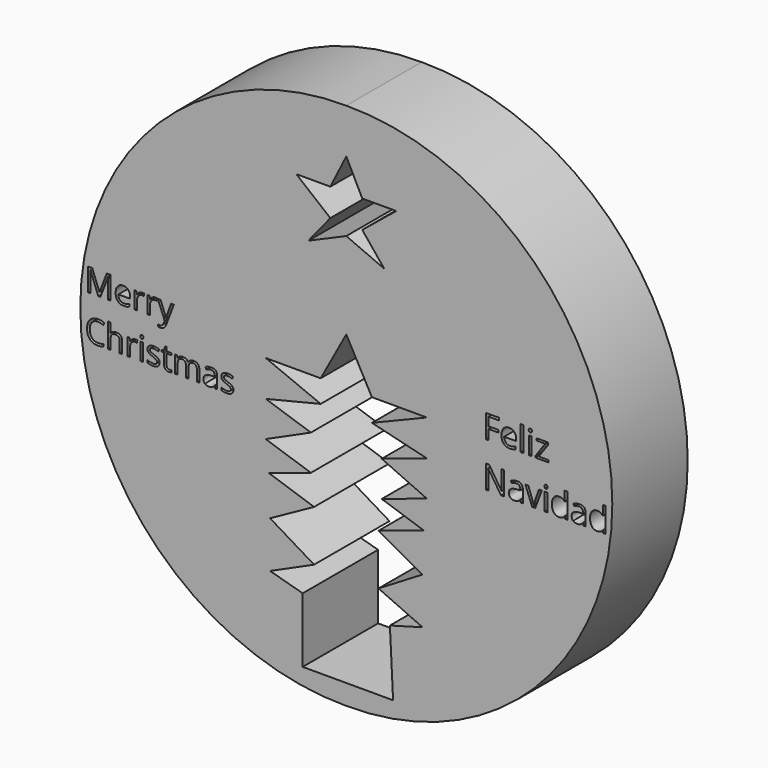
from build123d import *

# Parameters (mm, degrees)
F0_W     = 0.6967988684
F0_H     = 4.5983354994
F0_W_2   = 0.7130679342
F0_H_2   = 4.7056987948
F0_H_3   = 6.6814053253
F1_DEPTH = 25.4


with BuildPart() as f1:
    # F0 (on Front) → F1 (new body)
    with BuildSketch(Plane.XZ):
        with BuildLine():
            ThreePointArc((0, -75.4838734865), (71.6859873909, -4.2729414999), (0, 66.9379904866))
            ThreePointArc((0, 66.9379904866), (-71.6859873909, -4.2729414999), (0, -75.4838734865))
        make_face()
        with BuildLine():
            add(Edge.make_bspline(
                [(-65.5339630569, -6.4282716412), (-66.2307619253, -6.1020247722), (-66.9275607937, -6.1020247722)],
                knots=[0, 0, 0, 1, 1, 1], degree=2))
            add(Edge.make_bspline(
                [(-66.9275607937, -6.1020247722), (-67.9385233137, -6.1020247722), (-68.5238880663, -6.7753284957)],
                knots=[0, 0, 0, 1, 1, 1], degree=2))
            add(Edge.make_bspline(
                [(-68.5238880663, -6.7753284957), (-69.1092528189, -7.4486322192), (-69.1092528189, -8.6193617244)],
                knots=[0, 0, 0, 1, 1, 1], degree=2))
            add(Edge.make_bspline(
                [(-69.1092528189, -8.6193617244), (-69.1092528189, -9.8223131426), (-68.5446980518, -10.4795059096)],
                knots=[0, 0, 0, 1, 1, 1], degree=2))
            add(Edge.make_bspline(
                [(-68.5446980518, -10.4795059096), (-67.9801432846, -11.1366986766), (-66.9356162719, -11.1366986766)],
                knots=[0, 0, 0, 1, 1, 1], degree=2))
            add(Edge.make_bspline(
                [(-66.9356162719, -11.1366986766), (-66.2938631716, -11.1366986766), (-65.4708618106, -10.9057749669)],
                knots=[0, 0, 0, 1, 1, 1], degree=2))
            Line((-65.4708618106, -10.9057749669), (-65.4708618106, -11.530074531))
            add(Edge.make_bspline(
                [(-65.4708618106, -11.530074531), (-66.1085871719, -11.7703962987), (-67.0443652283, -11.7703962987)],
                knots=[0, 0, 0, 1, 1, 1], degree=2))
            add(Edge.make_bspline(
                [(-67.0443652283, -11.7703962987), (-68.3990281535, -11.7703962987), (-69.1354331232, -10.9473949378)],
                knots=[0, 0, 0, 1, 1, 1], degree=2))
            add(Edge.make_bspline(
                [(-69.1354331232, -10.9473949378), (-69.871838093, -10.1243935769), (-69.871838093, -8.6099636665)],
                knots=[0, 0, 0, 1, 1, 1], degree=2))
            add(Edge.make_bspline(
                [(-69.871838093, -8.6099636665), (-69.871838093, -7.6621023927), (-69.5173970501, -6.9491925678)],
                knots=[0, 0, 0, 1, 1, 1], degree=2))
            add(Edge.make_bspline(
                [(-69.5173970501, -6.9491925678), (-69.1629560072, -6.236282743), (-68.4936800229, -5.850291077)],
                knots=[0, 0, 0, 1, 1, 1], degree=2))
            add(Edge.make_bspline(
                [(-68.4936800229, -5.850291077), (-67.8244040385, -5.464299411), (-66.9181627357, -5.464299411)],
                knots=[0, 0, 0, 1, 1, 1], degree=2))
            add(Edge.make_bspline(
                [(-66.9181627357, -5.464299411), (-65.9541905055, -5.464299411), (-65.2318826227, -5.8160552944)],
                knots=[0, 0, 0, 1, 1, 1], degree=2))
            Line((-65.2318826227, -5.8160552944), (-65.5339630569, -6.4282716412))
        make_face(mode=Mode.SUBTRACT)
        with BuildLine():
            add(Edge.make_bspline(
                [(-57.6583904907, -7.2465739731), (-57.2972365492, -7.0028957562), (-56.8649258833, -7.0028957562)],
                knots=[0, 0, 0, 1, 1, 1], degree=2))
            add(Edge.make_bspline(
                [(-56.8649258833, -7.0028957562), (-56.5588177099, -7.0028957562), (-56.3158107828, -7.0539137851)],
                knots=[0, 0, 0, 1, 1, 1], degree=2))
            Line((-56.3158107828, -7.0539137851), (-56.4124765218, -7.6996946245))
            add(Edge.make_bspline(
                [(-56.4124765218, -7.6996946245), (-56.6971034198, -7.6365933783), (-56.9159439122, -7.6365933783)],
                knots=[0, 0, 0, 1, 1, 1], degree=2))
            add(Edge.make_bspline(
                [(-56.9159439122, -7.6365933783), (-57.4744570707, -7.6365933783), (-57.8705180845, -8.0897140297)],
                knots=[0, 0, 0, 1, 1, 1], degree=2))
            add(Edge.make_bspline(
                [(-57.8705180845, -8.0897140297), (-58.2665790983, -8.5428346811), (-58.2665790983, -9.2181522741)],
                knots=[0, 0, 0, 1, 1, 1], degree=2))
            Line((-58.2665790983, -9.2181522741), (-58.2665790983, -11.6858137771))
            Line((-58.2665790983, -11.6858137771), (-58.9633779667, -11.6858137771))
            Line((-58.9633779667, -11.6858137771), (-58.9633779667, -7.0874782778))
            Line((-58.9633779667, -7.0874782778), (-58.3887538517, -7.0874782778))
            Line((-58.3887538517, -7.0874782778), (-58.3081990693, -7.9386738125))
            Line((-58.3081990693, -7.9386738125), (-58.2746345766, -7.9386738125))
            add(Edge.make_bspline(
                [(-58.2746345766, -7.9386738125), (-58.0195444321, -7.4902521901), (-57.6583904907, -7.2465739731)],
                knots=[0, 0, 0, 1, 1, 1], degree=2))
        make_face(mode=Mode.SUBTRACT)
        with Locations((-55.1068177559, -9.3866460274)):
            Rectangle(F0_W, F0_H, mode=Mode.SUBTRACT)
        with BuildLine():
            Line((-60.3932253556, -11.6858137771), (-61.0900242239, -11.6858137771))
            Line((-61.0900242239, -11.6858137771), (-61.0900242239, -8.7106571445))
            add(Edge.make_bspline(
                [(-61.0900242239, -8.7106571445), (-61.0900242239, -8.1494588267), (-61.3457856583, -7.872216117)],
                knots=[0, 0, 0, 1, 1, 1], degree=2))
            add(Edge.make_bspline(
                [(-61.3457856583, -7.872216117), (-61.6015470926, -7.5949734073), (-62.1479770337, -7.5949734073)],
                knots=[0, 0, 0, 1, 1, 1], degree=2))
            add(Edge.make_bspline(
                [(-62.1479770337, -7.5949734073), (-62.872970076, -7.5949734073), (-63.2066011334, -7.9896918414)],
                knots=[0, 0, 0, 1, 1, 1], degree=2))
            add(Edge.make_bspline(
                [(-63.2066011334, -7.9896918414), (-63.5402321908, -8.3844102755), (-63.5402321908, -9.2812535204)],
                knots=[0, 0, 0, 1, 1, 1], degree=2))
            Line((-63.5402321908, -9.2812535204), (-63.5402321908, -11.6858137771))
            Line((-63.5402321908, -11.6858137771), (-64.2370310591, -11.6858137771))
            Line((-64.2370310591, -11.6858137771), (-64.2370310591, -5.1568486579))
            Line((-64.2370310591, -5.1568486579), (-63.5402321908, -5.1568486579))
            Line((-63.5402321908, -5.1568486579), (-63.5402321908, -7.1331259878))
            add(Edge.make_bspline(
                [(-63.5402321908, -7.1331259878), (-63.5402321908, -7.4902521901), (-63.5737966835, -7.725203639)],
                knots=[0, 0, 0, 1, 1, 1], degree=2))
            Line((-63.5737966835, -7.725203639), (-63.5321767125, -7.725203639))
            add(Edge.make_bspline(
                [(-63.5321767125, -7.725203639), (-63.3267620172, -7.3935864511), (-62.9468119599, -7.2029401326)],
                knots=[0, 0, 0, 1, 1, 1], degree=2))
            add(Edge.make_bspline(
                [(-62.9468119599, -7.2029401326), (-62.5668619026, -7.0122938141), (-62.0808480483, -7.0122938141)],
                knots=[0, 0, 0, 1, 1, 1], degree=2))
            add(Edge.make_bspline(
                [(-62.0808480483, -7.0122938141), (-61.2377079918, -7.0122938141), (-60.8154666737, -7.4130538569)],
                knots=[0, 0, 0, 1, 1, 1], degree=2))
            add(Edge.make_bspline(
                [(-60.8154666737, -7.4130538569), (-60.3932253556, -7.8138138997), (-60.3932253556, -8.6864907098)],
                knots=[0, 0, 0, 1, 1, 1], degree=2))
            Line((-60.3932253556, -8.6864907098), (-60.3932253556, -11.6858137771))
        make_face(mode=Mode.SUBTRACT)
        with BuildLine():
            add(Edge.make_bspline(
                [(-55.3968149728, -6.1919776126), (-55.5142906972, -6.0765157577), (-55.5142906972, -5.8415643089)],
                knots=[0, 0, 0, 1, 1, 1], degree=2))
            add(Edge.make_bspline(
                [(-55.5142906972, -5.8415643089), (-55.5142906972, -5.6025851209), (-55.3968149728, -5.4911510051)],
                knots=[0, 0, 0, 1, 1, 1], degree=2))
            add(Edge.make_bspline(
                [(-55.3968149728, -5.4911510051), (-55.2793392483, -5.3797168894), (-55.1021187269, -5.3797168894)],
                knots=[0, 0, 0, 1, 1, 1], degree=2))
            add(Edge.make_bspline(
                [(-55.1021187269, -5.3797168894), (-54.9342962634, -5.3797168894), (-54.8127927999, -5.4931648747)],
                knots=[0, 0, 0, 1, 1, 1], degree=2))
            add(Edge.make_bspline(
                [(-54.8127927999, -5.4931648747), (-54.6912893363, -5.60661286), (-54.6912893363, -5.8415643089)],
                knots=[0, 0, 0, 1, 1, 1], degree=2))
            add(Edge.make_bspline(
                [(-54.6912893363, -5.8415643089), (-54.6912893363, -6.0765157577), (-54.8127927999, -6.1919776126)],
                knots=[0, 0, 0, 1, 1, 1], degree=2))
            add(Edge.make_bspline(
                [(-54.8127927999, -6.1919776126), (-54.9342962634, -6.3074394675), (-55.1021187269, -6.3074394675)],
                knots=[0, 0, 0, 1, 1, 1], degree=2))
            add(Edge.make_bspline(
                [(-55.1021187269, -6.3074394675), (-55.2793392483, -6.3074394675), (-55.3968149728, -6.1919776126)],
                knots=[0, 0, 0, 1, 1, 1], degree=2))
        make_face(mode=Mode.SUBTRACT)
        with BuildLine():
            add(Edge.make_bspline(
                [(-50.6031341259, -9.6719442154), (-50.3158220684, -9.9740246496), (-50.3158220684, -10.43184433)],
                knots=[0, 0, 0, 1, 1, 1], degree=2))
            add(Edge.make_bspline(
                [(-50.3158220684, -10.43184433), (-50.3158220684, -11.0735974304), (-50.7937804444, -11.4219968645)],
                knots=[0, 0, 0, 1, 1, 1], degree=2))
            add(Edge.make_bspline(
                [(-50.7937804444, -11.4219968645), (-51.2717388204, -11.7703962987), (-52.1363601523, -11.7703962987)],
                knots=[0, 0, 0, 1, 1, 1], degree=2))
            add(Edge.make_bspline(
                [(-52.1363601523, -11.7703962987), (-53.0506569333, -11.7703962987), (-53.562179802, -11.4803990818)],
                knots=[0, 0, 0, 1, 1, 1], degree=2))
            Line((-53.562179802, -11.4803990818), (-53.562179802, -10.8346182424))
            add(Edge.make_bspline(
                [(-53.562179802, -10.8346182424), (-53.2305626142, -11.0024407058), (-52.8512838467, -11.098435155)],
                knots=[0, 0, 0, 1, 1, 1], degree=2))
            add(Edge.make_bspline(
                [(-52.8512838467, -11.098435155), (-52.4720050792, -11.1944296041), (-52.1189066161, -11.1944296041)],
                knots=[0, 0, 0, 1, 1, 1], degree=2))
            add(Edge.make_bspline(
                [(-52.1189066161, -11.1944296041), (-51.5738192547, -11.1944296041), (-51.2804655885, -11.0205655319)],
                knots=[0, 0, 0, 1, 1, 1], degree=2))
            add(Edge.make_bspline(
                [(-51.2804655885, -11.0205655319), (-50.9871119223, -10.8467014597), (-50.9871119223, -10.4895752574)],
                knots=[0, 0, 0, 1, 1, 1], degree=2))
            add(Edge.make_bspline(
                [(-50.9871119223, -10.4895752574), (-50.9871119223, -10.2210593159), (-51.2193782118, -10.0304129974)],
                knots=[0, 0, 0, 1, 1, 1], degree=2))
            add(Edge.make_bspline(
                [(-51.2193782118, -10.0304129974), (-51.4516445013, -9.8397666788), (-52.128304674, -9.5793062155)],
                knots=[0, 0, 0, 1, 1, 1], degree=2))
            add(Edge.make_bspline(
                [(-52.128304674, -9.5793062155), (-52.7700577744, -9.3403270275), (-53.0405875855, -9.1617639264)],
                knots=[0, 0, 0, 1, 1, 1], degree=2))
            add(Edge.make_bspline(
                [(-53.0405875855, -9.1617639264), (-53.3111173966, -8.9832008252), (-53.4433614979, -8.7569761445)],
                knots=[0, 0, 0, 1, 1, 1], degree=2))
            add(Edge.make_bspline(
                [(-53.4433614979, -8.7569761445), (-53.5756055991, -8.5307514637), (-53.5756055991, -8.2165878121)],
                knots=[0, 0, 0, 1, 1, 1], degree=2))
            add(Edge.make_bspline(
                [(-53.5756055991, -8.2165878121), (-53.5756055991, -7.6540469145), (-53.1177859187, -7.3284713353)],
                knots=[0, 0, 0, 1, 1, 1], degree=2))
            add(Edge.make_bspline(
                [(-53.1177859187, -7.3284713353), (-52.6599662383, -7.0028957562), (-51.8638164716, -7.0028957562)],
                knots=[0, 0, 0, 1, 1, 1], degree=2))
            add(Edge.make_bspline(
                [(-51.8638164716, -7.0028957562), (-51.1213698931, -7.0028957562), (-50.4111452277, -7.3049761904)],
                knots=[0, 0, 0, 1, 1, 1], degree=2))
            Line((-50.4111452277, -7.3049761904), (-50.6595224736, -7.8715448271))
            add(Edge.make_bspline(
                [(-50.6595224736, -7.8715448271), (-51.3509510232, -7.5869179291), (-51.9134919208, -7.5869179291)],
                knots=[0, 0, 0, 1, 1, 1], degree=2))
            add(Edge.make_bspline(
                [(-51.9134919208, -7.5869179291), (-52.408903833, -7.5869179291), (-52.6606375282, -7.7419858853)],
                knots=[0, 0, 0, 1, 1, 1], degree=2))
            add(Edge.make_bspline(
                [(-52.6606375282, -7.7419858853), (-52.9123712234, -7.8970538416), (-52.9123712234, -8.1695975223)],
                knots=[0, 0, 0, 1, 1, 1], degree=2))
            add(Edge.make_bspline(
                [(-52.9123712234, -8.1695975223), (-52.9123712234, -8.354873522), (-52.817719354, -8.4844324638)],
                knots=[0, 0, 0, 1, 1, 1], degree=2))
            add(Edge.make_bspline(
                [(-52.817719354, -8.4844324638), (-52.7230674846, -8.6139914056), (-52.5136250502, -8.73146713)],
                knots=[0, 0, 0, 1, 1, 1], degree=2))
            add(Edge.make_bspline(
                [(-52.5136250502, -8.73146713), (-52.3041826157, -8.8489428545), (-51.7080772255, -9.071811086)],
                knots=[0, 0, 0, 1, 1, 1], degree=2))
            add(Edge.make_bspline(
                [(-51.7080772255, -9.071811086), (-50.8904461834, -9.3698637811), (-50.6031341259, -9.6719442154)],
                knots=[0, 0, 0, 1, 1, 1], degree=2))
        make_face(mode=Mode.SUBTRACT)
        with BuildLine():
            add(Edge.make_bspline(
                [(-48.2388512604, -10.9722326624), (-48.0414920433, -11.1944296041), (-47.6977916381, -11.1944296041)],
                knots=[0, 0, 0, 1, 1, 1], degree=2))
            add(Edge.make_bspline(
                [(-47.6977916381, -11.1944296041), (-47.5125156384, -11.1944296041), (-47.3406654358, -11.1675780099)],
                knots=[0, 0, 0, 1, 1, 1], degree=2))
            add(Edge.make_bspline(
                [(-47.3406654358, -11.1675780099), (-47.1688152332, -11.1407264158), (-47.0681217551, -11.1111896622)],
                knots=[0, 0, 0, 1, 1, 1], degree=2))
            Line((-47.0681217551, -11.1111896622), (-47.0681217551, -11.6441938062))
            add(Edge.make_bspline(
                [(-47.0681217551, -11.6441938062), (-47.1808984506, -11.6978969945), (-47.4010815227, -11.7341466466)],
                knots=[0, 0, 0, 1, 1, 1], degree=2))
            add(Edge.make_bspline(
                [(-47.4010815227, -11.7341466466), (-47.6212645948, -11.7703962987), (-47.7984851162, -11.7703962987)],
                knots=[0, 0, 0, 1, 1, 1], degree=2))
            add(Edge.make_bspline(
                [(-47.7984851162, -11.7703962987), (-49.1316667661, -11.7703962987), (-49.1316667661, -10.3647153446)],
                knots=[0, 0, 0, 1, 1, 1], degree=2))
            Line((-49.1316667661, -10.3647153446), (-49.1316667661, -7.6285379))
            Line((-49.1316667661, -7.6285379), (-49.7908734026, -7.6285379))
            Line((-49.7908734026, -7.6285379), (-49.7908734026, -7.2928929731))
            Line((-49.7908734026, -7.2928929731), (-49.1316667661, -7.0028957562))
            Line((-49.1316667661, -7.0028957562), (-48.8389843898, -6.0214699897))
            Line((-48.8389843898, -6.0214699897), (-48.4362104774, -6.0214699897))
            Line((-48.4362104774, -6.0214699897), (-48.4362104774, -7.0874782778))
            Line((-48.4362104774, -7.0874782778), (-47.1016862478, -7.0874782778))
            Line((-47.1016862478, -7.0874782778), (-47.1016862478, -7.6285379))
            Line((-47.1016862478, -7.6285379), (-48.4362104774, -7.6285379))
            Line((-48.4362104774, -7.6285379), (-48.4362104774, -10.335178591))
            add(Edge.make_bspline(
                [(-48.4362104774, -10.335178591), (-48.4362104774, -10.7500357208), (-48.2388512604, -10.9722326624)],
                knots=[0, 0, 0, 1, 1, 1], degree=2))
        make_face(mode=Mode.SUBTRACT)
        with BuildLine():
            Line((-39.5926379418, -11.6858137771), (-40.2880942305, -11.6858137771))
            Line((-40.2880942305, -11.6858137771), (-40.2880942305, -8.694546188))
            add(Edge.make_bspline(
                [(-40.2880942305, -8.694546188), (-40.2880942305, -8.1440885078), (-40.5230456793, -7.8695309576)],
                knots=[0, 0, 0, 1, 1, 1], degree=2))
            add(Edge.make_bspline(
                [(-40.5230456793, -7.8695309576), (-40.7579971282, -7.5949734073), (-41.2534090404, -7.5949734073)],
                knots=[0, 0, 0, 1, 1, 1], degree=2))
            add(Edge.make_bspline(
                [(-41.2534090404, -7.5949734073), (-41.903217619, -7.5949734073), (-42.2140248214, -7.9682105661)],
                knots=[0, 0, 0, 1, 1, 1], degree=2))
            add(Edge.make_bspline(
                [(-42.2140248214, -7.9682105661), (-42.5248320238, -8.3414477249), (-42.5248320238, -9.117458796)],
                knots=[0, 0, 0, 1, 1, 1], degree=2))
            Line((-42.5248320238, -9.117458796), (-42.5248320238, -11.6858137771))
            Line((-42.5248320238, -11.6858137771), (-43.2216308921, -11.6858137771))
            Line((-43.2216308921, -11.6858137771), (-43.2216308921, -8.694546188))
            add(Edge.make_bspline(
                [(-43.2216308921, -8.694546188), (-43.2216308921, -8.1440885078), (-43.456582341, -7.8695309576)],
                knots=[0, 0, 0, 1, 1, 1], degree=2))
            add(Edge.make_bspline(
                [(-43.456582341, -7.8695309576), (-43.6915337899, -7.5949734073), (-44.1909734412, -7.5949734073)],
                knots=[0, 0, 0, 1, 1, 1], degree=2))
            add(Edge.make_bspline(
                [(-44.1909734412, -7.5949734073), (-44.8448097589, -7.5949734073), (-45.1489040627, -7.987006682)],
                knots=[0, 0, 0, 1, 1, 1], degree=2))
            add(Edge.make_bspline(
                [(-45.1489040627, -7.987006682), (-45.4529983666, -8.3790399567), (-45.4529983666, -9.2731980421)],
                knots=[0, 0, 0, 1, 1, 1], degree=2))
            Line((-45.4529983666, -9.2731980421), (-45.4529983666, -11.6858137771))
            Line((-45.4529983666, -11.6858137771), (-46.149797235, -11.6858137771))
            Line((-46.149797235, -11.6858137771), (-46.149797235, -7.0874782778))
            Line((-46.149797235, -7.0874782778), (-45.5832285982, -7.0874782778))
            Line((-45.5832285982, -7.0874782778), (-45.4704519028, -7.7171481607))
            Line((-45.4704519028, -7.7171481607), (-45.4368874101, -7.7171481607))
            add(Edge.make_bspline(
                [(-45.4368874101, -7.7171481607), (-45.239528193, -7.3815032338), (-44.8803881212, -7.192199495)],
                knots=[0, 0, 0, 1, 1, 1], degree=2))
            add(Edge.make_bspline(
                [(-44.8803881212, -7.192199495), (-44.5212480493, -7.0028957562), (-44.076854166, -7.0028957562)],
                knots=[0, 0, 0, 1, 1, 1], degree=2))
            add(Edge.make_bspline(
                [(-44.076854166, -7.0028957562), (-42.9987626606, -7.0028957562), (-42.6671454728, -7.7842771461)],
                knots=[0, 0, 0, 1, 1, 1], degree=2))
            Line((-42.6671454728, -7.7842771461), (-42.6335809801, -7.7842771461))
            add(Edge.make_bspline(
                [(-42.6335809801, -7.7842771461), (-42.4281662848, -7.4231232047), (-42.0381468797, -7.2130094804)],
                knots=[0, 0, 0, 1, 1, 1], degree=2))
            add(Edge.make_bspline(
                [(-42.0381468797, -7.2130094804), (-41.6481274745, -7.0028957562), (-41.1486878232, -7.0028957562)],
                knots=[0, 0, 0, 1, 1, 1], degree=2))
            add(Edge.make_bspline(
                [(-41.1486878232, -7.0028957562), (-40.3686490129, -7.0028957562), (-39.9806434774, -7.4036557989)],
                knots=[0, 0, 0, 1, 1, 1], degree=2))
            add(Edge.make_bspline(
                [(-39.9806434774, -7.4036557989), (-39.5926379418, -7.8044158417), (-39.5926379418, -8.6864907098)],
                knots=[0, 0, 0, 1, 1, 1], degree=2))
            Line((-39.5926379418, -8.6864907098), (-39.5926379418, -11.6858137771))
        make_face(mode=Mode.SUBTRACT)
        with BuildLine():
            Line((-34.8130541819, -11.6858137771), (-35.3299473694, -11.6858137771))
            Line((-35.3299473694, -11.6858137771), (-35.4682330793, -11.0306348797))
            Line((-35.4682330793, -11.0306348797), (-35.501797572, -11.0306348797))
            add(Edge.make_bspline(
                [(-35.501797572, -11.0306348797), (-35.8454979772, -11.4629455456), (-36.1871845128, -11.6166709222)],
                knots=[0, 0, 0, 1, 1, 1], degree=2))
            add(Edge.make_bspline(
                [(-36.1871845128, -11.6166709222), (-36.5288710485, -11.7703962987), (-37.0417364969, -11.7703962987)],
                knots=[0, 0, 0, 1, 1, 1], degree=2))
            add(Edge.make_bspline(
                [(-37.0417364969, -11.7703962987), (-37.7251095682, -11.7703962987), (-38.1131151038, -11.4172978356)],
                knots=[0, 0, 0, 1, 1, 1], degree=2))
            add(Edge.make_bspline(
                [(-38.1131151038, -11.4172978356), (-38.5011206393, -11.0641993724), (-38.5011206393, -10.4143907938)],
                knots=[0, 0, 0, 1, 1, 1], degree=2))
            add(Edge.make_bspline(
                [(-38.5011206393, -10.4143907938), (-38.5011206393, -9.0221356368), (-36.273780904, -8.9550066514)],
                knots=[0, 0, 0, 1, 1, 1], degree=2))
            Line((-36.273780904, -8.9550066514), (-35.4937420937, -8.9294976369))
            Line((-35.4937420937, -8.9294976369), (-35.4937420937, -8.6435281592))
            add(Edge.make_bspline(
                [(-35.4937420937, -8.6435281592), (-35.4937420937, -8.1024685369), (-35.7260083832, -7.844693233)],
                knots=[0, 0, 0, 1, 1, 1], degree=2))
            add(Edge.make_bspline(
                [(-35.7260083832, -7.844693233), (-35.9582746726, -7.5869179291), (-36.471140121, -7.5869179291)],
                knots=[0, 0, 0, 1, 1, 1], degree=2))
            add(Edge.make_bspline(
                [(-36.471140121, -7.5869179291), (-37.045764236, -7.5869179291), (-37.7707572782, -7.9386738125)],
                knots=[0, 0, 0, 1, 1, 1], degree=2))
            Line((-37.7707572782, -7.9386738125), (-37.9855700315, -7.4056696685))
            add(Edge.make_bspline(
                [(-37.9855700315, -7.4056696685), (-37.6458973654, -7.2217362485), (-37.2411095835, -7.1170150313)],
                knots=[0, 0, 0, 1, 1, 1], degree=2))
            add(Edge.make_bspline(
                [(-37.2411095835, -7.1170150313), (-36.8363218016, -7.0122938141), (-36.4281775704, -7.0122938141)],
                knots=[0, 0, 0, 1, 1, 1], degree=2))
            add(Edge.make_bspline(
                [(-36.4281775704, -7.0122938141), (-35.6065187892, -7.0122938141), (-35.2097864855, -7.3768042048)],
                knots=[0, 0, 0, 1, 1, 1], degree=2))
            add(Edge.make_bspline(
                [(-35.2097864855, -7.3768042048), (-34.8130541819, -7.7413145955), (-34.8130541819, -8.5468624202)],
                knots=[0, 0, 0, 1, 1, 1], degree=2))
            Line((-34.8130541819, -8.5468624202), (-34.8130541819, -11.6858137771))
        make_face(mode=Mode.SUBTRACT)
        with BuildLine():
            add(Edge.make_bspline(
                [(-30.7007325367, -9.6719442154), (-30.4134204792, -9.9740246496), (-30.4134204792, -10.43184433)],
                knots=[0, 0, 0, 1, 1, 1], degree=2))
            add(Edge.make_bspline(
                [(-30.4134204792, -10.43184433), (-30.4134204792, -11.0735974304), (-30.8913788552, -11.4219968645)],
                knots=[0, 0, 0, 1, 1, 1], degree=2))
            add(Edge.make_bspline(
                [(-30.8913788552, -11.4219968645), (-31.3693372312, -11.7703962987), (-32.2339585631, -11.7703962987)],
                knots=[0, 0, 0, 1, 1, 1], degree=2))
            add(Edge.make_bspline(
                [(-32.2339585631, -11.7703962987), (-33.1482553441, -11.7703962987), (-33.6597782128, -11.4803990818)],
                knots=[0, 0, 0, 1, 1, 1], degree=2))
            Line((-33.6597782128, -11.4803990818), (-33.6597782128, -10.8346182424))
            add(Edge.make_bspline(
                [(-33.6597782128, -10.8346182424), (-33.328161025, -11.0024407058), (-32.9488822575, -11.098435155)],
                knots=[0, 0, 0, 1, 1, 1], degree=2))
            add(Edge.make_bspline(
                [(-32.9488822575, -11.098435155), (-32.56960349, -11.1944296041), (-32.2165050269, -11.1944296041)],
                knots=[0, 0, 0, 1, 1, 1], degree=2))
            add(Edge.make_bspline(
                [(-32.2165050269, -11.1944296041), (-31.6714176655, -11.1944296041), (-31.3780639993, -11.0205655319)],
                knots=[0, 0, 0, 1, 1, 1], degree=2))
            add(Edge.make_bspline(
                [(-31.3780639993, -11.0205655319), (-31.0847103331, -10.8467014597), (-31.0847103331, -10.4895752574)],
                knots=[0, 0, 0, 1, 1, 1], degree=2))
            add(Edge.make_bspline(
                [(-31.0847103331, -10.4895752574), (-31.0847103331, -10.2210593159), (-31.3169766226, -10.0304129974)],
                knots=[0, 0, 0, 1, 1, 1], degree=2))
            add(Edge.make_bspline(
                [(-31.3169766226, -10.0304129974), (-31.5492429121, -9.8397666788), (-32.2259030848, -9.5793062155)],
                knots=[0, 0, 0, 1, 1, 1], degree=2))
            add(Edge.make_bspline(
                [(-32.2259030848, -9.5793062155), (-32.8676561852, -9.3403270275), (-33.1381859963, -9.1617639264)],
                knots=[0, 0, 0, 1, 1, 1], degree=2))
            add(Edge.make_bspline(
                [(-33.1381859963, -9.1617639264), (-33.4087158074, -8.9832008252), (-33.5409599087, -8.7569761445)],
                knots=[0, 0, 0, 1, 1, 1], degree=2))
            add(Edge.make_bspline(
                [(-33.5409599087, -8.7569761445), (-33.6732040099, -8.5307514637), (-33.6732040099, -8.2165878121)],
                knots=[0, 0, 0, 1, 1, 1], degree=2))
            add(Edge.make_bspline(
                [(-33.6732040099, -8.2165878121), (-33.6732040099, -7.6540469145), (-33.2153843295, -7.3284713353)],
                knots=[0, 0, 0, 1, 1, 1], degree=2))
            add(Edge.make_bspline(
                [(-33.2153843295, -7.3284713353), (-32.7575646491, -7.0028957562), (-31.9614148824, -7.0028957562)],
                knots=[0, 0, 0, 1, 1, 1], degree=2))
            add(Edge.make_bspline(
                [(-31.9614148824, -7.0028957562), (-31.2189683039, -7.0028957562), (-30.5087436385, -7.3049761904)],
                knots=[0, 0, 0, 1, 1, 1], degree=2))
            Line((-30.5087436385, -7.3049761904), (-30.7571208844, -7.8715448271))
            add(Edge.make_bspline(
                [(-30.7571208844, -7.8715448271), (-31.448549434, -7.5869179291), (-32.0110903316, -7.5869179291)],
                knots=[0, 0, 0, 1, 1, 1], degree=2))
            add(Edge.make_bspline(
                [(-32.0110903316, -7.5869179291), (-32.5065022438, -7.5869179291), (-32.758235939, -7.7419858853)],
                knots=[0, 0, 0, 1, 1, 1], degree=2))
            add(Edge.make_bspline(
                [(-32.758235939, -7.7419858853), (-33.0099696342, -7.8970538416), (-33.0099696342, -8.1695975223)],
                knots=[0, 0, 0, 1, 1, 1], degree=2))
            add(Edge.make_bspline(
                [(-33.0099696342, -8.1695975223), (-33.0099696342, -8.354873522), (-32.9153177648, -8.4844324638)],
                knots=[0, 0, 0, 1, 1, 1], degree=2))
            add(Edge.make_bspline(
                [(-32.9153177648, -8.4844324638), (-32.8206658954, -8.6139914056), (-32.611223461, -8.73146713)],
                knots=[0, 0, 0, 1, 1, 1], degree=2))
            add(Edge.make_bspline(
                [(-32.611223461, -8.73146713), (-32.4017810265, -8.8489428545), (-31.8056756363, -9.071811086)],
                knots=[0, 0, 0, 1, 1, 1], degree=2))
            add(Edge.make_bspline(
                [(-31.8056756363, -9.071811086), (-30.9880445942, -9.3698637811), (-30.7007325367, -9.6719442154)],
                knots=[0, 0, 0, 1, 1, 1], degree=2))
        make_face(mode=Mode.SUBTRACT)
        Polygon((-6.9040547602, 0), (0, 12.6621080562), (6.9040547602, 0), (21.6928608716, 0), (6.9040547602, -6.0824553717), (21.6928608716, -9.6894809976), (9.5448591746, -13.7388147414), (21.6928608716, -19.2343406379), (9.5448591746, -23.2836743817), (20.8251462318, -27.0437700674), (8.6771445349, -31.0931038111), (20.5335076898, -37.6447625458), (8.6771445349, -44.7868555784), (20.5335076898, -50.1434206963), (11.7491101846, -52.5841323872), (12.6087544486, -70.0391754508), (-11.7491101846, -70.0391754508), (-11.7491101846, -52.5841323872), (-20.5335076898, -50.1434206963), (-8.6771445349, -44.7868555784), (-20.5335076898, -37.6447625458), (-8.6771445349, -31.0931038111), (-20.8251462318, -27.0437700674), (-9.5448591746, -23.2836743817), (-21.6928608716, -19.2343406379), (-9.5448591746, -13.7388147414), (-21.6928608716, -9.6894809976), (-6.9040547602, -6.0824553717), (-21.6928608716, 0), align=None, mode=Mode.SUBTRACT)
        with BuildLine():
            Line((42.5357863907, -5.6811867201), (42.5357863907, -11.9586576087))
            Line((42.5357863907, -11.9586576087), (41.7031868375, -11.9586576087))
            Line((41.7031868375, -11.9586576087), (38.272491979, -6.6910228118))
            Line((38.272491979, -6.6910228118), (38.2381438126, -6.6910228118))
            add(Edge.make_bspline(
                [(38.2381438126, -6.6910228118), (38.3068401453, -7.6184233042), (38.3068401453, -8.3905700846)],
                knots=[0, 0, 0, 1, 1, 1], degree=2))
            Line((38.3068401453, -8.3905700846), (38.3068401453, -11.9586576087))
            Line((38.3068401453, -11.9586576087), (37.6322421575, -11.9586576087))
            Line((37.6322421575, -11.9586576087), (37.6322421575, -5.6811867201))
            Line((37.6322421575, -5.6811867201), (38.4565981508, -5.6811867201))
            Line((38.4565981508, -5.6811867201), (41.8790494494, -10.9282126171))
            Line((41.8790494494, -10.9282126171), (41.9133976158, -10.9282126171))
            add(Edge.make_bspline(
                [(41.9133976158, -10.9282126171), (41.9051540559, -10.8128027781), (41.8749276694, -10.1835443699)],
                knots=[0, 0, 0, 1, 1, 1], degree=2))
            add(Edge.make_bspline(
                [(41.8749276694, -10.1835443699), (41.844701283, -9.5542859617), (41.852944843, -9.2836224106)],
                knots=[0, 0, 0, 1, 1, 1], degree=2))
            Line((41.852944843, -9.2836224106), (41.852944843, -5.6811867201))
            Line((41.852944843, -5.6811867201), (42.5357863907, -5.6811867201))
        make_face(mode=Mode.SUBTRACT)
        with BuildLine():
            Line((47.5767232894, -11.9586576087), (47.0477615271, -11.9586576087))
            Line((47.0477615271, -11.9586576087), (46.9062470816, -11.2881814008))
            Line((46.9062470816, -11.2881814008), (46.8718989152, -11.2881814008))
            add(Edge.make_bspline(
                [(46.8718989152, -11.2881814008), (46.5201736914, -11.7305857839), (46.1705093576, -11.8879003859)],
                knots=[0, 0, 0, 1, 1, 1], degree=2))
            add(Edge.make_bspline(
                [(46.1705093576, -11.8879003859), (45.8208450238, -12.045214988), (45.2960050414, -12.045214988)],
                knots=[0, 0, 0, 1, 1, 1], degree=2))
            add(Edge.make_bspline(
                [(45.2960050414, -12.045214988), (44.5966763738, -12.045214988), (44.1996115704, -11.6838722776)],
                knots=[0, 0, 0, 1, 1, 1], degree=2))
            add(Edge.make_bspline(
                [(44.1996115704, -11.6838722776), (43.802546767, -11.3225295672), (43.802546767, -10.657549066)],
                knots=[0, 0, 0, 1, 1, 1], degree=2))
            add(Edge.make_bspline(
                [(43.802546767, -10.657549066), (43.802546767, -9.2327871243), (46.0818910883, -9.1640907916)],
                knots=[0, 0, 0, 1, 1, 1], degree=2))
            Line((46.0818910883, -9.1640907916), (46.8801424751, -9.1379861851))
            Line((46.8801424751, -9.1379861851), (46.8801424751, -8.8453398075))
            add(Edge.make_bspline(
                [(46.8801424751, -8.8453398075), (46.8801424751, -8.2916473654), (46.6424531637, -8.0278534476)],
                knots=[0, 0, 0, 1, 1, 1], degree=2))
            add(Edge.make_bspline(
                [(46.6424531637, -8.0278534476), (46.4047638523, -7.7640595297), (45.87992387, -7.7640595297)],
                knots=[0, 0, 0, 1, 1, 1], degree=2))
            add(Edge.make_bspline(
                [(45.87992387, -7.7640595297), (45.2918832614, -7.7640595297), (44.5499628675, -8.1240283134)],
                knots=[0, 0, 0, 1, 1, 1], degree=2))
            Line((44.5499628675, -8.1240283134), (44.3301346027, -7.5785794312))
            add(Edge.make_bspline(
                [(44.3301346027, -7.5785794312), (44.6777380465, -7.3903514794), (45.0919769331, -7.2831852003)],
                knots=[0, 0, 0, 1, 1, 1], degree=2))
            add(Edge.make_bspline(
                [(45.0919769331, -7.2831852003), (45.5062158197, -7.1760189212), (45.9238895229, -7.1760189212)],
                knots=[0, 0, 0, 1, 1, 1], degree=2))
            add(Edge.make_bspline(
                [(45.9238895229, -7.1760189212), (46.764732636, -7.1760189212), (47.1707279627, -7.5490400081)],
                knots=[0, 0, 0, 1, 1, 1], degree=2))
            add(Edge.make_bspline(
                [(47.1707279627, -7.5490400081), (47.5767232894, -7.9220610951), (47.5767232894, -8.7464170883)],
                knots=[0, 0, 0, 1, 1, 1], degree=2))
            Line((47.5767232894, -8.7464170883), (47.5767232894, -11.9586576087))
        make_face(mode=Mode.SUBTRACT)
        with BuildLine():
            Line((50.9071215021, -11.9586576087), (50.0745219489, -11.9586576087))
            Line((50.0745219489, -11.9586576087), (48.2884172969, -7.2529588139))
            Line((48.2884172969, -7.2529588139), (49.0523205173, -7.2529588139))
            Line((49.0523205173, -7.2529588139), (50.066278389, -10.043403851))
            add(Edge.make_bspline(
                [(50.066278389, -10.043403851), (50.4097600528, -11.0230135563), (50.4702128257, -11.3142860073)],
                knots=[0, 0, 0, 1, 1, 1], degree=2))
            Line((50.4702128257, -11.3142860073), (50.5045609921, -11.3142860073))
            add(Edge.make_bspline(
                [(50.5045609921, -11.3142860073), (50.5512744984, -11.0875881091), (50.8027030763, -10.372459285)],
                knots=[0, 0, 0, 1, 1, 1], degree=2))
            add(Edge.make_bspline(
                [(50.8027030763, -10.372459285), (51.0541316542, -9.6573304609), (51.9293229337, -7.2529588139)],
                knots=[0, 0, 0, 1, 1, 1], degree=2))
            Line((51.9293229337, -7.2529588139), (52.6932261541, -7.2529588139))
            Line((52.6932261541, -7.2529588139), (50.9071215021, -11.9586576087))
        make_face(mode=Mode.SUBTRACT)
        with Locations((53.8054197817, -9.6058082113)):
            Rectangle(F0_W_2, F0_H_2, mode=Mode.SUBTRACT)
        with BuildLine():
            Line((64.4842647109, -11.9586576087), (63.9553029485, -11.9586576087))
            Line((63.9553029485, -11.9586576087), (63.813788503, -11.2881814008))
            Line((63.813788503, -11.2881814008), (63.7794403366, -11.2881814008))
            add(Edge.make_bspline(
                [(63.7794403366, -11.2881814008), (63.4277151128, -11.7305857839), (63.078050779, -11.8879003859)],
                knots=[0, 0, 0, 1, 1, 1], degree=2))
            add(Edge.make_bspline(
                [(63.078050779, -11.8879003859), (62.7283864452, -12.045214988), (62.2035464629, -12.045214988)],
                knots=[0, 0, 0, 1, 1, 1], degree=2))
            add(Edge.make_bspline(
                [(62.2035464629, -12.045214988), (61.5042177953, -12.045214988), (61.1071529919, -11.6838722776)],
                knots=[0, 0, 0, 1, 1, 1], degree=2))
            add(Edge.make_bspline(
                [(61.1071529919, -11.6838722776), (60.7100881884, -11.3225295672), (60.7100881884, -10.657549066)],
                knots=[0, 0, 0, 1, 1, 1], degree=2))
            add(Edge.make_bspline(
                [(60.7100881884, -10.657549066), (60.7100881884, -9.2327871243), (62.9894325098, -9.1640907916)],
                knots=[0, 0, 0, 1, 1, 1], degree=2))
            Line((62.9894325098, -9.1640907916), (63.7876838966, -9.1379861851))
            Line((63.7876838966, -9.1379861851), (63.7876838966, -8.8453398075))
            add(Edge.make_bspline(
                [(63.7876838966, -8.8453398075), (63.7876838966, -8.2916473654), (63.5499945852, -8.0278534476)],
                knots=[0, 0, 0, 1, 1, 1], degree=2))
            add(Edge.make_bspline(
                [(63.5499945852, -8.0278534476), (63.3123052738, -7.7640595297), (62.7874652914, -7.7640595297)],
                knots=[0, 0, 0, 1, 1, 1], degree=2))
            add(Edge.make_bspline(
                [(62.7874652914, -7.7640595297), (62.1994246829, -7.7640595297), (61.457504289, -8.1240283134)],
                knots=[0, 0, 0, 1, 1, 1], degree=2))
            Line((61.457504289, -8.1240283134), (61.2376760241, -7.5785794312))
            add(Edge.make_bspline(
                [(61.2376760241, -7.5785794312), (61.5852794679, -7.3903514794), (61.9995183545, -7.2831852003)],
                knots=[0, 0, 0, 1, 1, 1], degree=2))
            add(Edge.make_bspline(
                [(61.9995183545, -7.2831852003), (62.4137572412, -7.1760189212), (62.8314309444, -7.1760189212)],
                knots=[0, 0, 0, 1, 1, 1], degree=2))
            add(Edge.make_bspline(
                [(62.8314309444, -7.1760189212), (63.6722740575, -7.1760189212), (64.0782693842, -7.5490400081)],
                knots=[0, 0, 0, 1, 1, 1], degree=2))
            add(Edge.make_bspline(
                [(64.0782693842, -7.5490400081), (64.4842647109, -7.9220610951), (64.4842647109, -8.7464170883)],
                knots=[0, 0, 0, 1, 1, 1], degree=2))
            Line((64.4842647109, -8.7464170883), (64.4842647109, -11.9586576087))
        make_face(mode=Mode.SUBTRACT)
        with BuildLine():
            Line((58.9706970427, -11.9586576087), (58.8758961035, -11.3280252738))
            Line((58.8758961035, -11.3280252738), (58.8374261571, -11.3280252738))
            add(Edge.make_bspline(
                [(58.8374261571, -11.3280252738), (58.3441864878, -12.045214988), (57.3604550026, -12.045214988)],
                knots=[0, 0, 0, 1, 1, 1], degree=2))
            add(Edge.make_bspline(
                [(57.3604550026, -12.045214988), (56.4371762901, -12.045214988), (55.9240146843, -11.4138956898)],
                knots=[0, 0, 0, 1, 1, 1], degree=2))
            add(Edge.make_bspline(
                [(55.9240146843, -11.4138956898), (55.4108530785, -10.7825763916), (55.4108530785, -9.6188605145)],
                knots=[0, 0, 0, 1, 1, 1], degree=2))
            add(Edge.make_bspline(
                [(55.4108530785, -9.6188605145), (55.4108530785, -8.4551446374), (55.9260755743, -7.810773036)],
                knots=[0, 0, 0, 1, 1, 1], degree=2))
            add(Edge.make_bspline(
                [(55.9260755743, -7.810773036), (56.4412980701, -7.1664014346), (57.3604550026, -7.1664014346)],
                knots=[0, 0, 0, 1, 1, 1], degree=2))
            add(Edge.make_bspline(
                [(57.3604550026, -7.1664014346), (58.3180818814, -7.1664014346), (58.8291825972, -7.8629822489)],
                knots=[0, 0, 0, 1, 1, 1], degree=2))
            Line((58.8291825972, -7.8629822489), (58.8855135901, -7.8629822489))
            Line((58.8855135901, -7.8629822489), (58.8552872036, -7.523622365))
            Line((58.8552872036, -7.523622365), (58.8374261571, -7.1925060411))
            Line((58.8374261571, -7.1925060411), (58.8374261571, -5.2772522834))
            Line((58.8374261571, -5.2772522834), (59.5504940913, -5.2772522834))
            Line((59.5504940913, -5.2772522834), (59.5504940913, -11.9586576087))
            Line((59.5504940913, -11.9586576087), (58.9706970427, -11.9586576087))
        make_face(mode=Mode.SUBTRACT)
        with BuildLine():
            add(Edge.make_bspline(
                [(53.5086516241, -6.3365497347), (53.3884330418, -6.2183920424), (53.3884330418, -5.9779548777)],
                knots=[0, 0, 0, 1, 1, 1], degree=2))
            add(Edge.make_bspline(
                [(53.3884330418, -5.9779548777), (53.3884330418, -5.733395933), (53.5086516241, -5.6193600206)],
                knots=[0, 0, 0, 1, 1, 1], degree=2))
            add(Edge.make_bspline(
                [(53.5086516241, -5.6193600206), (53.6288702065, -5.5053241082), (53.810228525, -5.5053241082)],
                knots=[0, 0, 0, 1, 1, 1], degree=2))
            add(Edge.make_bspline(
                [(53.810228525, -5.5053241082), (53.9819693569, -5.5053241082), (54.1063097192, -5.6214209106)],
                knots=[0, 0, 0, 1, 1, 1], degree=2))
            add(Edge.make_bspline(
                [(54.1063097192, -5.6214209106), (54.2306500815, -5.737517713), (54.2306500815, -5.9779548777)],
                knots=[0, 0, 0, 1, 1, 1], degree=2))
            add(Edge.make_bspline(
                [(54.2306500815, -5.9779548777), (54.2306500815, -6.2183920424), (54.1063097192, -6.3365497347)],
                knots=[0, 0, 0, 1, 1, 1], degree=2))
            add(Edge.make_bspline(
                [(54.1063097192, -6.3365497347), (53.9819693569, -6.4547074271), (53.810228525, -6.4547074271)],
                knots=[0, 0, 0, 1, 1, 1], degree=2))
            add(Edge.make_bspline(
                [(53.810228525, -6.4547074271), (53.6288702065, -6.4547074271), (53.5086516241, -6.3365497347)],
                knots=[0, 0, 0, 1, 1, 1], degree=2))
        make_face(mode=Mode.SUBTRACT)
        with BuildLine():
            Line((69.2490423518, -11.9586576087), (69.1542414126, -11.3280252738))
            Line((69.1542414126, -11.3280252738), (69.1157714662, -11.3280252738))
            add(Edge.make_bspline(
                [(69.1157714662, -11.3280252738), (68.6225317969, -12.045214988), (67.6388003117, -12.045214988)],
                knots=[0, 0, 0, 1, 1, 1], degree=2))
            add(Edge.make_bspline(
                [(67.6388003117, -12.045214988), (66.7155215992, -12.045214988), (66.2023599934, -11.4138956898)],
                knots=[0, 0, 0, 1, 1, 1], degree=2))
            add(Edge.make_bspline(
                [(66.2023599934, -11.4138956898), (65.6891983876, -10.7825763916), (65.6891983876, -9.6188605145)],
                knots=[0, 0, 0, 1, 1, 1], degree=2))
            add(Edge.make_bspline(
                [(65.6891983876, -9.6188605145), (65.6891983876, -8.4551446374), (66.2044208834, -7.810773036)],
                knots=[0, 0, 0, 1, 1, 1], degree=2))
            add(Edge.make_bspline(
                [(66.2044208834, -7.810773036), (66.7196433792, -7.1664014346), (67.6388003117, -7.1664014346)],
                knots=[0, 0, 0, 1, 1, 1], degree=2))
            add(Edge.make_bspline(
                [(67.6388003117, -7.1664014346), (68.5964271905, -7.1664014346), (69.1075279063, -7.8629822489)],
                knots=[0, 0, 0, 1, 1, 1], degree=2))
            Line((69.1075279063, -7.8629822489), (69.1638588992, -7.8629822489))
            Line((69.1638588992, -7.8629822489), (69.1336325128, -7.523622365))
            Line((69.1336325128, -7.523622365), (69.1157714662, -7.1925060411))
            Line((69.1157714662, -7.1925060411), (69.1157714662, -5.2772522834))
            Line((69.1157714662, -5.2772522834), (69.8288394004, -5.2772522834))
            Line((69.8288394004, -5.2772522834), (69.8288394004, -11.9586576087))
            Line((69.8288394004, -11.9586576087), (69.2490423518, -11.9586576087))
        make_face(mode=Mode.SUBTRACT)
        with BuildLine():
            Line((-66.264326418, 0), (-66.838950533, 0))
            Line((-66.838950533, 0), (-68.9199490801, 5.4374478168))
            Line((-68.9199490801, 5.4374478168), (-68.9535135728, 5.4374478168))
            add(Edge.make_bspline(
                [(-68.9535135728, 5.4374478168), (-68.8944400657, 4.7916669773), (-68.8944400657, 3.901536631)],
                knots=[0, 0, 0, 1, 1, 1], degree=2))
            Line((-68.8944400657, 3.901536631), (-68.8944400657, 0))
            Line((-68.8944400657, 0), (-69.5536467022, 0))
            Line((-69.5536467022, 0), (-69.5536467022, 6.1342466852))
            Line((-69.5536467022, 6.1342466852), (-68.4795829359, 6.1342466852))
            Line((-68.4795829359, 6.1342466852), (-66.5368700987, 1.0740637663))
            Line((-66.5368700987, 1.0740637663), (-66.503305606, 1.0740637663))
            Line((-66.503305606, 1.0740637663), (-64.5444818122, 6.1342466852))
            Line((-64.5444818122, 6.1342466852), (-63.4784735242, 6.1342466852))
            Line((-63.4784735242, 6.1342466852), (-63.4784735242, 0))
            Line((-63.4784735242, 0), (-64.1913833491, 0))
            Line((-64.1913833491, 0), (-64.1913833491, 3.9525546599))
            add(Edge.make_bspline(
                [(-64.1913833491, 3.9525546599), (-64.1913833491, 4.6318999921), (-64.1323098419, 5.4293923386)],
                knots=[0, 0, 0, 1, 1, 1], degree=2))
            Line((-64.1323098419, 5.4293923386), (-64.1658743346, 5.4293923386))
            Line((-64.1658743346, 5.4293923386), (-66.264326418, 0))
        make_face(mode=Mode.SUBTRACT)
        with BuildLine():
            add(Edge.make_bspline(
                [(-59.1634223432, -0.0147683768), (-59.4923543716, -0.0845825216), (-59.9582295302, -0.0845825216)],
                knots=[0, 0, 0, 1, 1, 1], degree=2))
            add(Edge.make_bspline(
                [(-59.9582295302, -0.0845825216), (-60.9772475285, -0.0845825216), (-61.5673113101, 0.5370318831)],
                knots=[0, 0, 0, 1, 1, 1], degree=2))
            add(Edge.make_bspline(
                [(-61.5673113101, 0.5370318831), (-62.1573750917, 1.1586462879), (-62.1573750917, 2.260904228)],
                knots=[0, 0, 0, 1, 1, 1], degree=2))
            add(Edge.make_bspline(
                [(-62.1573750917, 2.260904228), (-62.1573750917, 3.3739028058), (-61.6096025709, 4.0284104134)],
                knots=[0, 0, 0, 1, 1, 1], degree=2))
            add(Edge.make_bspline(
                [(-61.6096025709, 4.0284104134), (-61.0618300501, 4.682918021), (-60.1381352111, 4.682918021)],
                knots=[0, 0, 0, 1, 1, 1], degree=2))
            add(Edge.make_bspline(
                [(-60.1381352111, 4.682918021), (-59.2748564589, 4.682918021), (-58.7713890685, 4.1143355147)],
                knots=[0, 0, 0, 1, 1, 1], degree=2))
            add(Edge.make_bspline(
                [(-58.7713890685, 4.1143355147), (-58.267921678, 3.5457530084), (-58.267921678, 2.6140026912)],
                knots=[0, 0, 0, 1, 1, 1], degree=2))
            Line((-58.267921678, 2.6140026912), (-58.267921678, 2.173636547))
            Line((-58.267921678, 2.173636547), (-61.4350672088, 2.173636547))
            add(Edge.make_bspline(
                [(-61.4350672088, 2.173636547), (-61.4135859335, 1.3640609832), (-61.025580398, 0.9445048245)],
                knots=[0, 0, 0, 1, 1, 1], degree=2))
            add(Edge.make_bspline(
                [(-61.025580398, 0.9445048245), (-60.6375748624, 0.5249486658), (-59.9327205158, 0.5249486658)],
                knots=[0, 0, 0, 1, 1, 1], degree=2))
            add(Edge.make_bspline(
                [(-59.9327205158, 0.5249486658), (-59.1902739373, 0.5249486658), (-58.4652808951, 0.8350845783)],
                knots=[0, 0, 0, 1, 1, 1], degree=2))
            Line((-58.4652808951, 0.8350845783), (-58.4652808951, 0.2134701735))
            add(Edge.make_bspline(
                [(-58.4652808951, 0.2134701735), (-58.8344903147, 0.055045768), (-59.1634223432, -0.0147683768)],
                knots=[0, 0, 0, 1, 1, 1], degree=2))
        make_face(mode=Mode.SUBTRACT)
        with BuildLine():
            add(Edge.make_bspline(
                [(-55.7747511605, 4.439239804), (-55.4135972191, 4.682918021), (-54.9812865532, 4.682918021)],
                knots=[0, 0, 0, 1, 1, 1], degree=2))
            add(Edge.make_bspline(
                [(-54.9812865532, 4.682918021), (-54.6751783798, 4.682918021), (-54.4321714527, 4.6318999921)],
                knots=[0, 0, 0, 1, 1, 1], degree=2))
            Line((-54.4321714527, 4.6318999921), (-54.5288371917, 3.9861191526))
            add(Edge.make_bspline(
                [(-54.5288371917, 3.9861191526), (-54.8134640897, 4.0492203989), (-55.0323045821, 4.0492203989)],
                knots=[0, 0, 0, 1, 1, 1], degree=2))
            add(Edge.make_bspline(
                [(-55.0323045821, 4.0492203989), (-55.5908177406, 4.0492203989), (-55.9868787544, 3.5960997475)],
                knots=[0, 0, 0, 1, 1, 1], degree=2))
            add(Edge.make_bspline(
                [(-55.9868787544, 3.5960997475), (-56.3829397682, 3.1429790961), (-56.3829397682, 2.467661503)],
                knots=[0, 0, 0, 1, 1, 1], degree=2))
            Line((-56.3829397682, 2.467661503), (-56.3829397682, 0))
            Line((-56.3829397682, 0), (-57.0797386366, 0))
            Line((-57.0797386366, 0), (-57.0797386366, 4.5983354994))
            Line((-57.0797386366, 4.5983354994), (-56.5051145216, 4.5983354994))
            Line((-56.5051145216, 4.5983354994), (-56.4245597391, 3.7471399646))
            Line((-56.4245597391, 3.7471399646), (-56.3909952464, 3.7471399646))
            add(Edge.make_bspline(
                [(-56.3909952464, 3.7471399646), (-56.135905102, 4.195561587), (-55.7747511605, 4.439239804)],
                knots=[0, 0, 0, 1, 1, 1], degree=2))
        make_face(mode=Mode.SUBTRACT)
        with BuildLine():
            add(Edge.make_bspline(
                [(-52.2665903839, 4.439239804), (-51.9054364425, 4.682918021), (-51.4731257766, 4.682918021)],
                knots=[0, 0, 0, 1, 1, 1], degree=2))
            add(Edge.make_bspline(
                [(-51.4731257766, 4.682918021), (-51.1670176032, 4.682918021), (-50.9240106761, 4.6318999921)],
                knots=[0, 0, 0, 1, 1, 1], degree=2))
            Line((-50.9240106761, 4.6318999921), (-51.020676415, 3.9861191526))
            add(Edge.make_bspline(
                [(-51.020676415, 3.9861191526), (-51.3053033131, 4.0492203989), (-51.5241438055, 4.0492203989)],
                knots=[0, 0, 0, 1, 1, 1], degree=2))
            add(Edge.make_bspline(
                [(-51.5241438055, 4.0492203989), (-52.082656964, 4.0492203989), (-52.4787179778, 3.5960997475)],
                knots=[0, 0, 0, 1, 1, 1], degree=2))
            add(Edge.make_bspline(
                [(-52.4787179778, 3.5960997475), (-52.8747789916, 3.1429790961), (-52.8747789916, 2.467661503)],
                knots=[0, 0, 0, 1, 1, 1], degree=2))
            Line((-52.8747789916, 2.467661503), (-52.8747789916, 0))
            Line((-52.8747789916, 0), (-53.57157786, 0))
            Line((-53.57157786, 0), (-53.57157786, 4.5983354994))
            Line((-53.57157786, 4.5983354994), (-52.996953745, 4.5983354994))
            Line((-52.996953745, 4.5983354994), (-52.9163989625, 3.7471399646))
            Line((-52.9163989625, 3.7471399646), (-52.8828344698, 3.7471399646))
            add(Edge.make_bspline(
                [(-52.8828344698, 3.7471399646), (-52.6277443253, 4.195561587), (-52.2665903839, 4.439239804)],
                knots=[0, 0, 0, 1, 1, 1], degree=2))
        make_face(mode=Mode.SUBTRACT)
        with BuildLine():
            Line((-48.9383352882, -0.0255090144), (-50.7937804444, 4.5983354994))
            Line((-50.7937804444, 4.5983354994), (-50.0459635471, 4.5983354994))
            Line((-50.0459635471, 4.5983354994), (-49.0390287663, 1.97627733))
            add(Edge.make_bspline(
                [(-49.0390287663, 1.97627733), (-48.7087541581, 1.0780915054), (-48.6281993756, 0.6793453322)],
                knots=[0, 0, 0, 1, 1, 1], degree=2))
            Line((-48.6281993756, 0.6793453322), (-48.594634883, 0.6793453322))
            add(Edge.make_bspline(
                [(-48.594634883, 0.6793453322), (-48.5409316946, 0.8941580854), (-48.3663963326, 1.4123938527)],
                knots=[0, 0, 0, 1, 1, 1], degree=2))
            add(Edge.make_bspline(
                [(-48.3663963326, 1.4123938527), (-48.1918609706, 1.9306296199), (-47.2265461607, 4.5983354994)],
                knots=[0, 0, 0, 1, 1, 1], degree=2))
            Line((-47.2265461607, 4.5983354994), (-46.4800718431, 4.5983354994))
            Line((-46.4800718431, 4.5983354994), (-48.456349173, -0.6377253612))
            add(Edge.make_bspline(
                [(-48.456349173, -0.6377253612), (-48.7503741291, -1.4137364324), (-49.1424074038, -1.7393120115)],
                knots=[0, 0, 0, 1, 1, 1], degree=2))
            add(Edge.make_bspline(
                [(-49.1424074038, -1.7393120115), (-49.5344406784, -2.0648875907), (-50.1050370543, -2.0648875907)],
                knots=[0, 0, 0, 1, 1, 1], degree=2))
            add(Edge.make_bspline(
                [(-50.1050370543, -2.0648875907), (-50.4245710248, -2.0648875907), (-50.7347069373, -1.9923882865)],
                knots=[0, 0, 0, 1, 1, 1], degree=2))
            Line((-50.7347069373, -1.9923882865), (-50.7347069373, -1.4352177077))
            add(Edge.make_bspline(
                [(-50.7347069373, -1.4352177077), (-50.5037832275, -1.4848931569), (-50.2191563295, -1.4848931569)],
                knots=[0, 0, 0, 1, 1, 1], degree=2))
            add(Edge.make_bspline(
                [(-50.2191563295, -1.4848931569), (-49.5008761858, -1.4848931569), (-49.1947680124, -0.6793453322)],
                knots=[0, 0, 0, 1, 1, 1], degree=2))
            Line((-49.1947680124, -0.6793453322), (-48.9383352882, -0.0255090144))
        make_face(mode=Mode.SUBTRACT)
        Polygon((38.3617972116, 2.683278758), (38.3617972116, 0), (37.6322421575, 0), (37.6322421575, 6.2774708886), (41.1316333489, 6.2774708886), (41.1316333489, 5.6289775072), (38.3617972116, 5.6289775072), (38.3617972116, 3.3317721394), (40.9640142969, 3.3317721394), (40.9640142969, 2.683278758), align=None, mode=Mode.SUBTRACT)
        with BuildLine():
            add(Edge.make_bspline(
                [(44.8645920716, -0.0151131932), (44.527980041, -0.0865573793), (44.0512274916, -0.0865573793)],
                knots=[0, 0, 0, 1, 1, 1], degree=2))
            add(Edge.make_bspline(
                [(44.0512274916, -0.0865573793), (43.0084171602, -0.0865573793), (42.4045763951, 0.5495706622)],
                knots=[0, 0, 0, 1, 1, 1], degree=2))
            add(Edge.make_bspline(
                [(42.4045763951, 0.5495706622), (41.8007356301, 1.1856987036), (41.8007356301, 2.3136924877)],
                knots=[0, 0, 0, 1, 1, 1], degree=2))
            add(Edge.make_bspline(
                [(41.8007356301, 2.3136924877), (41.8007356301, 3.452677685), (42.3612977055, 4.1224669296)],
                knots=[0, 0, 0, 1, 1, 1], degree=2))
            add(Edge.make_bspline(
                [(42.3612977055, 4.1224669296), (42.9218597809, 4.7922561741), (43.8671213198, 4.7922561741)],
                knots=[0, 0, 0, 1, 1, 1], degree=2))
            add(Edge.make_bspline(
                [(43.8671213198, 4.7922561741), (44.7505561592, 4.7922561741), (45.265778655, 4.2103982355)],
                knots=[0, 0, 0, 1, 1, 1], degree=2))
            add(Edge.make_bspline(
                [(45.265778655, 4.2103982355), (45.7810011508, 3.6285402969), (45.7810011508, 2.6750351981)],
                knots=[0, 0, 0, 1, 1, 1], degree=2))
            Line((45.7810011508, 2.6750351981), (45.7810011508, 2.2243872551))
            Line((45.7810011508, 2.2243872551), (42.5399081707, 2.2243872551))
            add(Edge.make_bspline(
                [(42.5399081707, 2.2243872551), (42.5618909971, 1.3959094819), (42.9589558006, 0.9665574021)],
                knots=[0, 0, 0, 1, 1, 1], degree=2))
            add(Edge.make_bspline(
                [(42.9589558006, 0.9665574021), (43.356020604, 0.5372053223), (44.0773320981, 0.5372053223)],
                knots=[0, 0, 0, 1, 1, 1], degree=2))
            add(Edge.make_bspline(
                [(44.0773320981, 0.5372053223), (44.8371135385, 0.5372053223), (45.5790339324, 0.8545823797)],
                knots=[0, 0, 0, 1, 1, 1], degree=2))
            Line((45.5790339324, 0.8545823797), (45.5790339324, 0.2184543382))
            add(Edge.make_bspline(
                [(45.5790339324, 0.2184543382), (45.2012041022, 0.0563309929), (44.8645920716, -0.0151131932)],
                knots=[0, 0, 0, 1, 1, 1], degree=2))
        make_face(mode=Mode.SUBTRACT)
        with Locations((47.3534602079, 3.3407026626)):
            Rectangle(F0_W_2, F0_H_3, mode=Mode.SUBTRACT)
        with Locations((49.577847463, 2.3528493974)):
            Rectangle(F0_W_2, F0_H_2, mode=Mode.SUBTRACT)
        Polygon((54.455974053, 0.5536924421), (54.455974053, 0), (51.0417663143, 0), (51.0417663143, 0.4849961094), (53.6096352333, 4.1520063526), (51.2011418064, 4.1520063526), (51.2011418064, 4.7056987948), (54.3913995002, 4.7056987948), (54.3913995002, 4.1520063526), (51.8578787476, 0.5536924421), align=None, mode=Mode.SUBTRACT)
        with BuildLine():
            add(Edge.make_bspline(
                [(49.2810793054, 5.6221078739), (49.1608607231, 5.7402655663), (49.1608607231, 5.980702731)],
                knots=[0, 0, 0, 1, 1, 1], degree=2))
            add(Edge.make_bspline(
                [(49.1608607231, 5.980702731), (49.1608607231, 6.2252616757), (49.2810793054, 6.3392975881)],
                knots=[0, 0, 0, 1, 1, 1], degree=2))
            add(Edge.make_bspline(
                [(49.2810793054, 6.3392975881), (49.4012978878, 6.4533335005), (49.5826562063, 6.4533335005)],
                knots=[0, 0, 0, 1, 1, 1], degree=2))
            add(Edge.make_bspline(
                [(49.5826562063, 6.4533335005), (49.7543970382, 6.4533335005), (49.8787374005, 6.3372366981)],
                knots=[0, 0, 0, 1, 1, 1], degree=2))
            add(Edge.make_bspline(
                [(49.8787374005, 6.3372366981), (50.0030777628, 6.2211398957), (50.0030777628, 5.980702731)],
                knots=[0, 0, 0, 1, 1, 1], degree=2))
            add(Edge.make_bspline(
                [(50.0030777628, 5.980702731), (50.0030777628, 5.7402655663), (49.8787374005, 5.6221078739)],
                knots=[0, 0, 0, 1, 1, 1], degree=2))
            add(Edge.make_bspline(
                [(49.8787374005, 5.6221078739), (49.7543970382, 5.5039501816), (49.5826562063, 5.5039501816)],
                knots=[0, 0, 0, 1, 1, 1], degree=2))
            add(Edge.make_bspline(
                [(49.5826562063, 5.5039501816), (49.4012978878, 5.5039501816), (49.2810793054, 5.6221078739)],
                knots=[0, 0, 0, 1, 1, 1], degree=2))
        make_face(mode=Mode.SUBTRACT)
        Polygon((-4.2984690517, 46.3054403663), (0, 54.9023337662), (4.2984690517, 46.3054403663), (13.4684881195, 46.3054403663), (4.2984690517, 38.8548001647), (10.2239194682, 31.5619378287), (0, 35.9891690314), (-10.2239194682, 31.5619378287), (-4.2984690517, 38.8548001647), (-13.4684881195, 46.3054403663), align=None, mode=Mode.SUBTRACT)
    extrude(amount=F1_DEPTH)


solid = f1.part
